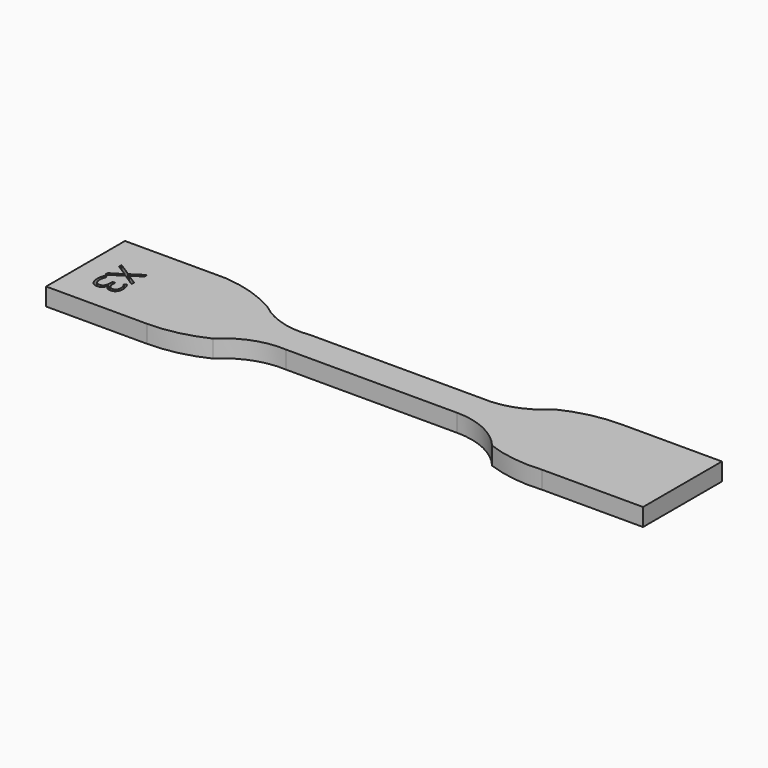
from build123d import *

# Parameters (mm, degrees)
F1_DEPTH     = 3.4
F2_TEXT_SIZE = 7.0564552314
F3_DEPTH     = 1


# Not quite as in the source:
# - Text() gives the source's letters only with a copy of the font that has no kerning and outlines rounded to 1/6400 em; it was checked with that copy


with BuildPart() as f1:
    # F0 (on Top) → F1 (new body)
    with BuildSketch(Plane.XY):
        with BuildLine():
            Line((-14.4320548165, 19.7811394548), (-33.8720548165, 19.7811394548))
            Line((-33.8720548165, 19.7811394548), (-33.8720548165, 0.7811394548))
            Line((-33.8720548165, 0.7811394548), (-14.4320548165, 0.7811394548))
            ThreePointArc((-14.4320548165, 0.7811394548), (-8.9053122052, 1.3996892086), (-3.6520548165, 3.2247301661))
            ThreePointArc((-3.6520548165, 3.2247301661), (1.3014698263, 6.4128780055), (7.1279451835, 7.2811394548))
            Line((7.1279451835, 7.2811394548), (40.1279451835, 7.2811394548))
            ThreePointArc((40.1279451835, 7.2811394548), (46.0837574042, 5.9511158081), (50.9079451835, 2.2137538538))
            ThreePointArc((50.9079451835, 2.2137538538), (56.2191047011, 0.9041953221), (61.6879451835, 0.7811394548))
            Line((61.6879451835, 0.7811394548), (81.1279451835, 0.7811394548))
            Line((81.1279451835, 0.7811394548), (81.1279451835, 19.7811394548))
            Line((81.1279451835, 19.7811394548), (61.6879451835, 19.7811394548))
            ThreePointArc((61.6879451835, 19.7811394548), (56.1612025723, 19.162589701), (50.9079451835, 17.3375487435))
            ThreePointArc((50.9079451835, 17.3375487435), (45.9544205407, 14.1494009041), (40.1279451835, 13.2811394548))
            Line((40.1279451835, 13.2811394548), (7.1279451835, 13.2811394548))
            ThreePointArc((7.1279451835, 13.2811394548), (1.4167452884, 13.6925537245), (-3.6520548165, 16.3560723447))
            ThreePointArc((-3.6520548165, 16.3560723447), (-8.8458057958, 18.686276846), (-14.4320548165, 19.7811394548))
        make_face()
    extrude(amount=F1_DEPTH)

    # F2 (on face) → F3 (cut)
    with BuildSketch(Plane.XY.offset(3.4)):
        with Locations(Location((-29.3720550835, 13.353464842), (0, 0, -90))):
            Text('X3', F2_TEXT_SIZE, font='Open Sans', text_align=(TextAlign.LEFT, TextAlign.BOTTOM))
    extrude(amount=-F3_DEPTH, mode=Mode.SUBTRACT)


solid = f1.part
